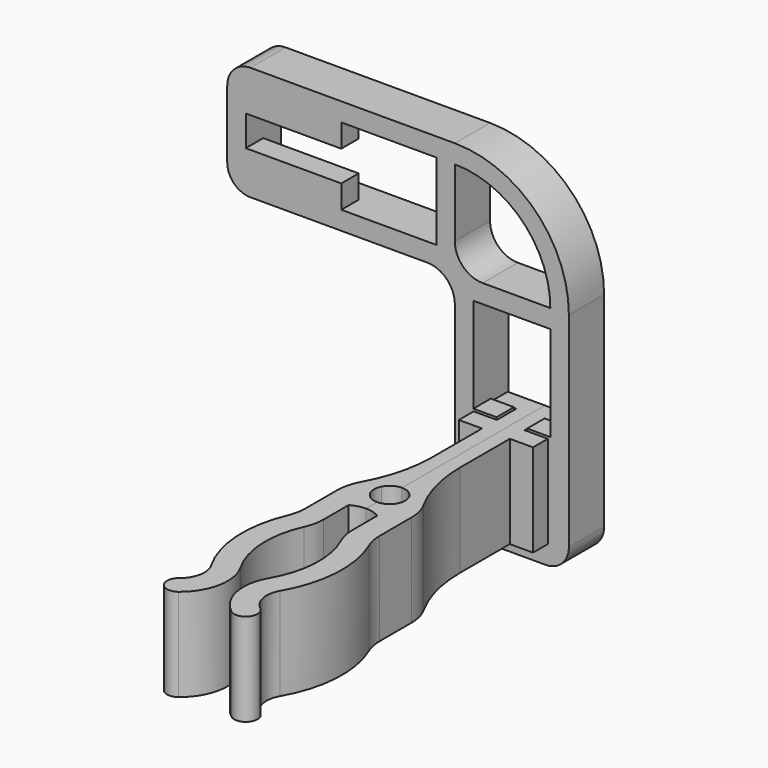
from build123d import *
from build123d import SkipClean  # not in build123d's __all__

# Parameters (mm, degrees)
F1_DEPTH = 20
F2_R     = 10
F6_DEPTH = 9.5
F5_W     = 20.6
F5_H     = 5
F5_W_2   = 5
F5_H_2   = 20.6
F7_DEPTH = 4.7
F8_R     = 5


with BuildPart() as f1:
    # F0 (on Top) → F1 (new body)
    with BuildSketch(Plane.XY):
        with BuildLine():
            Line((8, 0), (0, 0))
            Line((0, 0), (0, -4))
            Line((0, -4), (5, -4))
            Line((5, -4), (5, -9.2))
            Line((5, -9.2), (0, -9.2))
            Line((0, -9.2), (0, -13.2))
            Line((0, -13.2), (5, -13.2))
            Line((5, -13.2), (5, -26.6168760482))
            Line((5, -26.6168760482), (5, -40.3678421966))
            ThreePointArc((5, -40.3678421966), (6.234427286, -39.0088181315), (8, -38.5053202414))
            Line((8, -38.5053202414), (8, 0))
        make_face()
        with BuildLine():
            Line((8, -48.2), (8, -45.2))
            ThreePointArc((8, -45.2), (5.1561580109, -43.6182328347), (5, -40.3678421966))
            Line((5, -40.3678421966), (5, -26.6168760482))
            ThreePointArc((5, -26.6168760482), (3.7228132327, -35.2771300861), (0, -43.2))
            Line((0, -43.2), (0, -56.7436034959))
            ThreePointArc((0, -56.7436034959), (-2.7724216072, -68.7945299554), (0.5698729811, -80.7))
            ThreePointArc((0.5698729811, -80.7), (1.2008963786, -84.4594516542), (-0.7860771969, -87.7126966924))
            ThreePointArc((-0.7860771969, -87.7126966924), (-1.2100240798, -91.2227207722), (2.3, -91.6466676551))
            ThreePointArc((2.3, -91.6466676551), (6.109971325, -85.4086529871), (4.9, -78.2))
            ThreePointArc((4.9, -78.2), (2.2205080757, -68.2), (4.9, -58.2))
            Line((4.9, -58.2), (4.9, -49.0628801844))
            ThreePointArc((4.9, -49.0628801844), (6.3910747211, -48.4197439982), (8, -48.2))
        make_face()
    extrude(amount=F1_DEPTH)

    # F2
    f2_edges = [f1.edges().sort_by_distance(p)[0] for p in [
        (4.9, -58.2, 10),
        (0, -56.743603, 10),
        (0, -43.2, 10),
    ]]
    fillet(f2_edges, radius=F2_R)

    # F3: F1 across face


with BuildPart() as f1_1:
    add(f1.part, clean=False)
    with SkipClean():  # cleaning this boolean's faces spoils the solid; the shape is the same uncleaned
        add(f1.part.mirror(Plane(origin=(8, -19.2526601207, 10), x_dir=(0, 1, 0), z_dir=(1, 0, 0))), clean=False)


with BuildPart() as f6:
    # F5 (on offset) → F6 (new body)
    with BuildSketch(Plane(origin=(0, -8.9, 0), x_dir=(-1, 0, 0), z_dir=(0, 1, 0))):
        with BuildLine():
            Line((-20.3, -4.3), (4.3, -4.3))
            Line((4.3, -4.3), (4.3, 38.8))
            ThreePointArc((4.3, 38.8), (6.0573593129, 43.0426406871), (10.3, 44.8))
            Line((10.3, 44.8), (53.4, 44.8))
            Line((53.4, 44.8), (53.4, 69.4))
            Line((53.4, 69.4), (4.3, 69.4))
            ThreePointArc((4.3, 69.4), (-13.0948268172, 62.1948268172), (-20.3, 44.8))
            Line((-20.3, 44.8), (-20.3, -4.3))
        make_face()
        Polygon((0.3, -0.3), (-4.7, -0.3), (-11.3, -0.3), (-16.3, -0.3), (-16.3, 20.3), (-16.3, 40.8), (0.3, 40.8), (0.3, 20.3), align=None, mode=Mode.SUBTRACT)
        with BuildLine():
            ThreePointArc((4.3, 50.8), (2.5426406871, 46.5573593129), (-1.7, 44.8))
            Line((-1.7, 44.8), (-16.3, 44.8))
            ThreePointArc((-16.3, 44.8), (-10.2663996924, 59.3663996924), (4.3, 65.4))
            Line((4.3, 65.4), (4.3, 50.8))
        make_face(mode=Mode.SUBTRACT)
        Polygon((8.3, 65.4), (28.8, 65.4), (49.4, 65.4), (49.4, 60.4), (49.4, 53.8), (49.4, 48.8), (28.8, 48.8), (8.3, 48.8), align=None, mode=Mode.SUBTRACT)
    extrude(amount=F6_DEPTH)

    # F5 (on offset) → F7 (join)
    with BuildSketch(Plane(origin=(0, -8.9, 0), x_dir=(-1, 0, 0), z_dir=(0, 1, 0))):
        with Locations((39.1, 51.3)):
            Rectangle(F5_W, F5_H)
        with Locations((39.1, 62.9)):
            Rectangle(F5_W, F5_H)
        with Locations((-13.8, 10)):
            Rectangle(F5_W_2, F5_H_2)
        with Locations((-2.2, 10)):
            Rectangle(F5_W_2, F5_H_2)
    extrude(amount=F7_DEPTH)

    # F8
    f8_edges = [f6.edges().sort_by_distance(p)[0] for p in [
        (-53.4, -4.15, 44.8),
        (-53.4, -4.15, 69.4),
        (20.3, -4.15, -4.3),
        (-4.3, -4.15, -4.3),
    ]]
    fillet(f8_edges, radius=F8_R)


solid = Compound([f1_1.part, f6.part])
